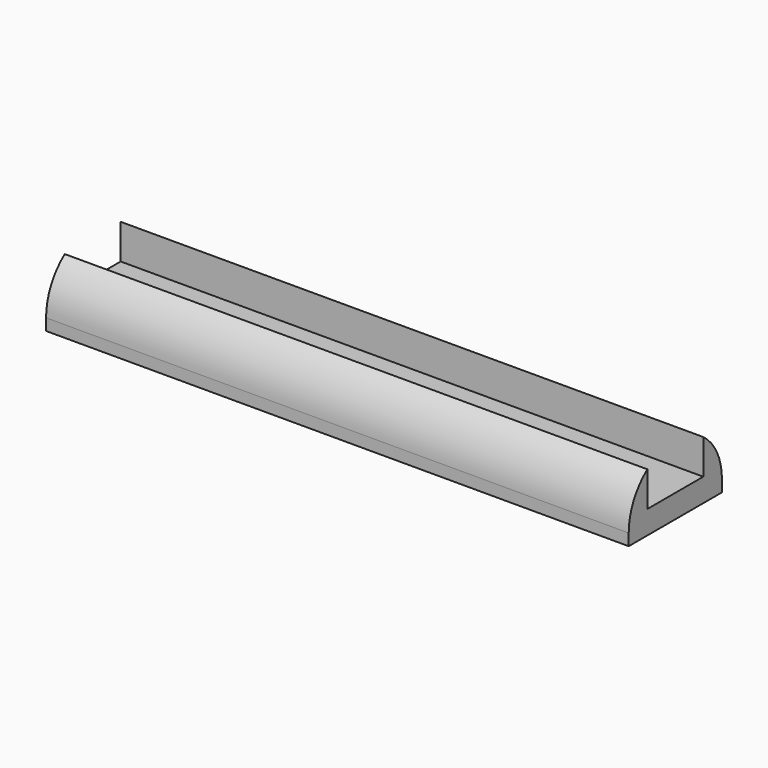
from build123d import *

# Parameters (mm, degrees)
F0_W        = 50
F0_H        = 6
F0_H_2      = 2
F1_DEPTH    = 2
F2_DEPTH    = 5
F3_T1_DEPTH = 70


# Not quite as in the source:
# - a fillet or chamfer that OpenCascade refuses, or shapes differently, is made with other operations: its cross-section is extruded or revolved along the edge and cut away or added
# - a feature names something its author has since deleted; it is built from what else it names


with BuildPart() as f1:
    # F0 (on Top) → F1 (new body)
    with BuildSketch(Plane.XY):
        Rectangle(F0_W, F0_H)
        with Locations((0, 4)):
            Rectangle(F0_W, F0_H_2)
        with Locations((0, -4)):
            Rectangle(F0_W, F0_H_2)
    extrude(amount=F1_DEPTH)

    # F0 (on Top) → F2 (join)
    with BuildSketch(Plane.XY):
        with Locations((0, 4)):
            Rectangle(F0_W, F0_H_2)
        with Locations((0, -4)):
            Rectangle(F0_W, F0_H_2)
    extrude(amount=F2_DEPTH)

    # F3: fillet of radius 5 on 2 edges, made by hand

    # F3_s2 → F3_t1 (cut)
    with BuildSketch(Plane.YZ.offset(-35)):
        with BuildLine():
            ThreePointArc((-5, 1), (-4.472135955, 3.2360679775), (-3, 5))
            Line((-3, 5), (-5, 5))
            Line((-5, 5), (-5, 1))
        make_face()
        with BuildLine():
            ThreePointArc((5, 1), (4.472135955, 3.2360679775), (3, 5))
            Line((3, 5), (5, 5))
            Line((5, 5), (5, 1))
        make_face()
    extrude(amount=F3_T1_DEPTH, mode=Mode.SUBTRACT)


solid = f1.part
